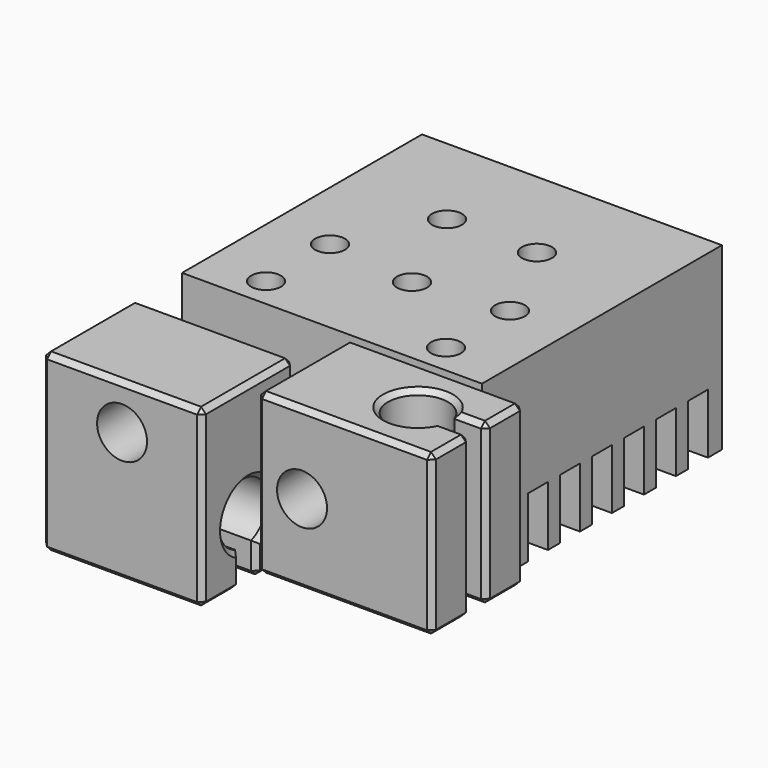
from build123d import *

# Parameters (mm, degrees)
F0_W      = 30
F0_H      = 30
F11_DEPTH = 18
F1_D      = 8
F1_DEPTH  = 6.5
F1_TIP    = 2.4034424761
F13_W     = 30
F13_H     = 2.5
F14_DEPTH = 6
F15_D     = 3
F15_DEPTH = 10
F15_TIP   = 0.9012909285
F2_R      = 1.475
F3_DEPTH  = 3.5
F17_W     = 16
F17_H     = 17.5
F16_W     = 17.5
F16_H     = 16
F18_DEPTH = 11.5
F5_DEPTH  = 16
F21_DEPTH = 16
F8_SIZE   = 0.5
F7_R      = 1.5
F9_DEPTH  = 8
F20_R     = 2.5
F19_R     = 2.5
F10_DEPTH = 6


# Not quite as in the source:
# - a feature names something its author has since deleted; it is built from what else it names


with BuildPart() as f11:
    # F0 (on Top) → F11 (new body)
    with BuildSketch(Plane.XY):
        Rectangle(F0_W, F0_H)
    extrude(amount=F11_DEPTH)

    # F1
    with Locations(Plane(origin=(0, 15, 0), x_dir=(-1, 0, 0), z_dir=(0, 1, 0))):
        with Locations((-9, 12), (9, 12)):
            Hole(F1_D / 2, depth=F1_DEPTH)
            with Locations((0, 0, -(F1_DEPTH + F1_TIP / 2))):  # 118° drill point
                Cone(0, F1_D / 2, F1_TIP, mode=Mode.SUBTRACT)

    # F13 (on face) → F14 (cut)
    with BuildSketch(Plane(origin=(0, 0, 0), x_dir=(1, 0, 0), z_dir=(0, 0, -1))):
        with Locations((0, 12)):
            Rectangle(F13_W, F13_H)
        with Locations((0, 8)):
            Rectangle(F13_W, F13_H)
        with Locations((0, 4)):
            Rectangle(F13_W, F13_H)
        Rectangle(F13_W, F13_H)
        with Locations((0, -4)):
            Rectangle(F13_W, F13_H)
        with Locations((0, -8)):
            Rectangle(F13_W, F13_H)
        with Locations((0, -12)):
            Rectangle(F13_W, F13_H)
    extrude(amount=-F14_DEPTH, mode=Mode.SUBTRACT)

    # F15
    with Locations(Plane(origin=(0, 15, 0), x_dir=(-1, 0, 0), z_dir=(0, 1, 0))):
        with Locations((8.5, 3), (-8.5, 3), (0, 15)):
            Hole(F15_D / 2, depth=F15_DEPTH)
            with Locations((0, 0, -(F15_DEPTH + F15_TIP / 2))):  # 118° drill point
                Cone(0, F15_D / 2, F15_TIP, mode=Mode.SUBTRACT)

    # F2 (on face) → F3 (join)
    with BuildSketch(Plane.XZ.offset(15)):
        with Locations((-9, 12)):
            Circle(F2_R)
        with Locations((9, 12)):
            Circle(F2_R)
    extrude(amount=F3_DEPTH)

    # F17 (on face) + F16 (on face) → F18 (join)
    with BuildSketch(Plane.XZ.offset(18.5)):
        with Locations((-9, 7.75)):
            Rectangle(F17_W, F17_H)
    with BuildSketch(Plane.XZ.offset(18.5)):
        with Locations((13.25, 12)):
            Rectangle(F16_W, F16_H)
    extrude(amount=F18_DEPTH)

    # F4 (on face) → F5 (cut, through all)
    with BuildSketch(Plane(origin=(0, 0, 4), x_dir=(1, 0, 0), z_dir=(0, 0, -1))):
        with BuildLine():
            Line((22, 25.25), (18.8284271247, 25.25))
            ThreePointArc((18.8284271247, 25.25), (13, 24.25), (18.8284271247, 23.25))
            Line((18.8284271247, 23.25), (22, 23.25))
            Line((22, 23.25), (22, 25.25))
        make_face()
    extrude(amount=-F5_DEPTH, mode=Mode.SUBTRACT)

    # F6 (on face) → F21 (cut, through all)
    with BuildSketch(Plane(origin=(-17, 0, 0), x_dir=(0, -1, 0), z_dir=(-1, 0, 0))):
        with BuildLine():
            Line((25.25, -1), (25.25, 2.1715728753))
            ThreePointArc((25.25, 2.1715728753), (24.25, 8), (23.25, 2.1715728753))
            Line((23.25, 2.1715728753), (23.25, -1))
            Line((23.25, -1), (25.25, -1))
        make_face()
    extrude(amount=-F21_DEPTH, mode=Mode.SUBTRACT)

    # F8
    f8_edges = [f11.edges().sort_by_distance(p)[0] for p in [
        (13.25, -18.5, 4),
        (22, -20.875, 4),
        (20.414214, -23.25, 4),
        (13, -24.25, 4),
        (20.414214, -25.25, 4),
        (22, -27.625, 4),
        (13.25, -30, 4),
        (4.5, -24.25, 4),
        (4.5, -24.25, 20),
        (4.5, -18.5, 12),
        (4.5, -30, 12),
        (-9, -25.25, -1),
        (-1, -27.625, -1),
        (-9, -30, -1),
        (-17, -27.625, -1),
        (-9, -18.5, -1),
        (-1, -20.875, -1),
        (-9, -23.25, -1),
        (-17, -20.875, -1),
        (-1, -18.5, 7.75),
        (-1, -24.25, 16.5),
        (-1, -30, 7.75),
        (-1, -25.25, 0.585786),
        (-1, -24.25, 8),
        (-1, -23.25, 0.585786),
        (22, -18.5, 12),
        (22, -20.875, 20),
        (22, -23.25, 12),
        (22, -25.25, 12),
        (22, -27.625, 20),
        (22, -30, 12),
        (-17, -24.25, 16.5),
        (-9, -18.5, 16.5),
        (-9, -30, 16.5),
        (-17, -18.5, 7.75),
        (-17, -23.25, 0.585786),
        (-17, -24.25, 8),
        (-17, -25.25, 0.585786),
        (-17, -30, 7.75),
        (13.25, -18.5, 20),
        (13.25, -30, 20),
        (20.414214, -25.25, 20),
        (13, -24.25, 20),
        (20.414214, -23.25, 20),
    ]]
    chamfer(f8_edges, length=F8_SIZE)

    # F7 (on face) → F9 (cut)
    with BuildSketch(Plane.XY.offset(18)):
        with Locations((-9, -12)):
            Circle(F7_R)
        with Locations((-9, -4)):
            Circle(F7_R)
        with Locations((0, -5)):
            Circle(F7_R)
        with Locations((4.5, 5)):
            Circle(F7_R)
        with Locations((9, -4)):
            Circle(F7_R)
        with Locations((9, -12)):
            Circle(F7_R)
        with Locations((-4.5, 5)):
            Circle(F7_R)
    extrude(amount=-F9_DEPTH, mode=Mode.SUBTRACT)

    # F20 (on face) + F19 (on face) → F10 (cut)
    with BuildSketch(Plane.XZ.offset(30)):
        with Locations((-9, 12)):
            Circle(F20_R)
    with BuildSketch(Plane.XZ.offset(30)):
        with Locations((9, 12)):
            Circle(F19_R)
    extrude(amount=-F10_DEPTH, mode=Mode.SUBTRACT)


solid = f11.part
